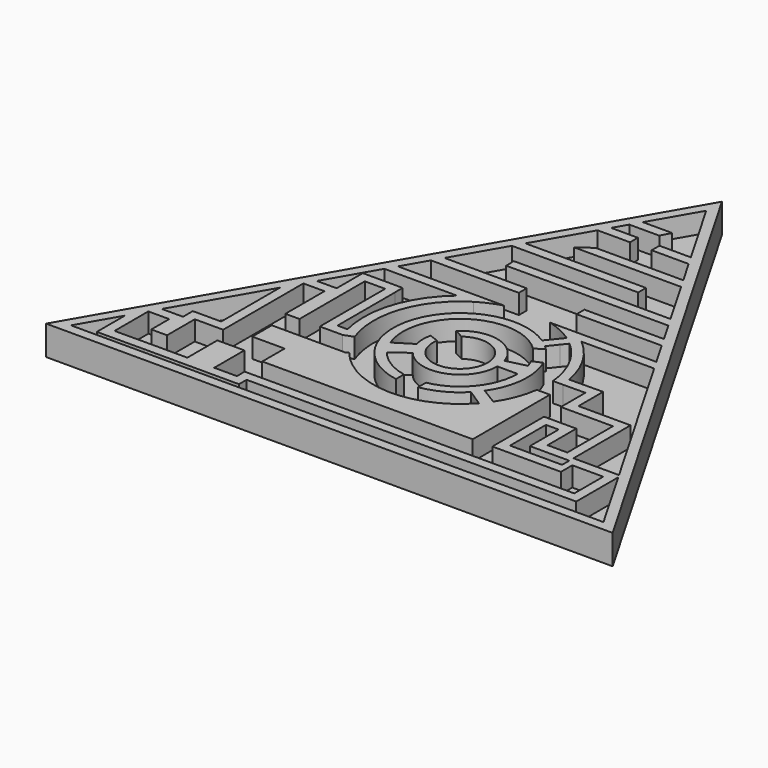
from build123d import *

# Parameters (mm, degrees)
F1_DEPTH = 4
F3_DEPTH = 2


# Not quite as in the source:
# - ends of sketch curves that miss each other by under 0.0002 mm in the source are joined


with BuildPart() as f1:
    # F0 (on Top) → F1 (new body)
    with BuildSketch(Plane.XY):
        Polygon((57.7278355129, -33.3416372538), (0, 66.6583627462), (-57.7278355129, -33.3416372538), align=None)
        Polygon((-36.4066096967, -6.9060390815), (-36.4066096967, -13.5858934373), (-36.4066096967, -15.3864606768), (-40.186252445, -15.3864606768), (-42.186252445, -15.3864606768), (-42.186252445, -17.3864606768), (-42.186252445, -17.8865476996), (-43.4002317488, -17.8865476996), (-46.4966176706, -17.8865476996), (-36.4066096967, -0.4079641283), align=None, mode=Mode.SUBTRACT)
        with BuildLine():
            Line((-27.4925772248, 15.0335163855), (-26.3380205146, 15.0335163855))
            Line((-26.3380205146, 15.0335163855), (-12.690151286, 15.0335163855))
            ThreePointArc((-12.690151286, 15.0335163855), (-18.7426502915, 5.9799343329), (-19.0519640748, -4.9060390815))
            Line((-19.0519640748, -4.9060390815), (-21.0900533497, -4.9060390815))
            Line((-21.0900533497, -4.9060390815), (-21.0900533497, 9.7259394825))
            Line((-21.0900533497, 9.7259394825), (-21.1140420288, 9.7259394825))
            Line((-21.1140420288, 9.7259394825), (-21.1140420288, 11.7116095498))
            Line((-21.1140420288, 11.7116095498), (-23.0900533497, 11.7116095498))
            Line((-23.0900533497, 11.7116095498), (-23.0900533497, 11.7259394825))
            Line((-23.0900533497, 11.7259394825), (-27.2341445088, 11.7259394825))
            Line((-27.2341445088, 11.7259394825), (-29.2341445088, 11.7259394825))
            Line((-29.2341445088, 11.7259394825), (-29.2341445088, 9.7259394825))
            Line((-29.2341445088, 9.7259394825), (-29.2341445088, 5.0565690249))
            Line((-29.2341445088, 5.0565690249), (-30.1103927195, 5.0565690249))
            Line((-30.1103927195, 5.0565690249), (-33.2520529864, 5.0565690249))
            Line((-33.2520529864, 5.0565690249), (-27.4925772248, 15.0335163855))
        make_face(mode=Mode.SUBTRACT)
        Polygon((54.2639496366, -31.3416372538), (-54.2639496366, -31.3416372538), (-49.6511743809, -23.3510808528), (-49.6511743809, -24.4550537318), (-49.6511743809, -28.5100210458), (-49.6511743809, -30.5099894606), (-47.6399342756, -30.5099894606), (-40.0851143612, -30.4675303044), (-40.0738744334, -30.4674671345), (-32.8411310911, -30.4674987197), (-27.3643452674, -30.4674987197), (-20.8822563291, -30.4674987197), (-20.7181237638, -30.4674987197), (-20.7181237638, -28.5053253174), (-20.7108877152, -28.525368914), (-12.9712559283, -28.525368914), (18.1306451559, -28.525368914), (46.4564595819, -28.525368914), (46.4564595819, -26.525368914), (46.4564595819, -19.1514473408), (46.4564595819, -17.8169831846), align=None, mode=Mode.SUBTRACT)
        Polygon((26.1836768538, -20.0500268042), (26.1836768538, -10.8962344453), (28.761634931, -10.8962344453), (28.761634931, -16.2106864154), (28.761634931, -18.2106864154), (30.761634931, -18.2106864154), (34.7944386303, -18.2106864154), (36.7944386303, -18.2106864154), (36.7944386303, -20.0500268042), align=None, mode=Mode.SUBTRACT)
        with BuildLine():
            ThreePointArc((19.3406121337, 3.6037864629), (17.0044739065, 9.8941609921), (12.690151286, 15.0335163855))
            Line((12.690151286, 15.0335163855), (26.3380205146, 15.0335163855))
            Line((26.3380205146, 15.0335163855), (27.4925772248, 15.0335163855))
            Line((27.4925772248, 15.0335163855), (46.0722601447, -17.1514473408))
            Line((46.0722601447, -17.1514473408), (44.4564595819, -17.1514473408))
            Line((44.4564595819, -17.1514473408), (38.1584949791, -17.1514473408))
            Line((38.1584949791, -17.1514473408), (36.7944386303, -17.1514473408))
            Line((36.7944386303, -17.1514473408), (36.7944386303, -16.2106864154))
            Line((36.7944386303, -16.2106864154), (36.7944386303, -8.8962344453))
            Line((36.7944386303, -8.8962344453), (36.7944386303, -2.6055312268))
            Line((36.7944386303, -2.6055312268), (26.1836768538, -2.6055312268))
            Line((26.1836768538, -2.6055312268), (26.1836768538, 3.6767962217))
            Line((26.1836768538, 3.6767962217), (19.456515533, 3.6019981121))
            Line((19.456515533, 3.6019981121), (19.3409452762, 3.6019981121))
            ThreePointArc((19.3409452762, 3.6019981121), (19.3407787256, 3.6028922914), (19.3406121337, 3.6037864629))
        make_face(mode=Mode.SUBTRACT)
        with BuildLine():
            Line((-5.4116371698, 53.2835908234), (0, 62.6579890175))
            Line((0, 62.6579890175), (8.1201158924, 48.5917836587))
            Line((8.1201158924, 48.5917836588), (1.7250510864, 48.5917836588))
            Line((1.7250510864, 48.5917836588), (1.7250510864, 46.5917824588))
            Line((1.7250510864, 46.5917824588), (8.1201158924, 46.5917824588))
            Line((8.1201158924, 46.5917824588), (9.2746732954, 46.5917824588))
            Line((9.2746732954, 46.5917824587), (12.115224579, 41.6711904109))
            Line((12.115224579, 41.6711904109), (-5.7159573771, 41.6711904109))
            Line((-5.7159573771, 41.6711904109), (-8.5862353444, 39.6711895109))
            Line((-8.5862353444, 39.6711895109), (12.0601376528, 39.6711895109))
            Line((12.0601376528, 39.6711895109), (13.2697818089, 39.6711895109))
            Line((13.2697818089, 39.6711895109), (18.8652666503, 29.9783181399))
            Line((18.8652666503, 29.9783181399), (-13.0685195327, 29.9783181399))
            Line((-13.0685195327, 29.9783181399), (-13.0114983767, 27.9783181399))
            Line((-13.0114983767, 27.9783181399), (18.7051940445, 27.9783181399))
            Line((18.7051940445, 27.9783181399), (20.0198233606, 27.9783181399))
            Line((20.0198233606, 27.9783181399), (22.353366566, 23.9359992401))
            Line((22.353366566, 23.9359992401), (6.1596790329, 23.9359992401))
            Line((6.1596790329, 23.9359992401), (6.1596790329, 21.9359992401))
            Line((6.1596790329, 21.9359992401), (22.353366566, 21.9359992401))
            Line((22.353366566, 21.9359992401), (23.5079232763, 21.9359992401))
            Line((23.5079232763, 21.9359992401), (26.3380205146, 17.0335163855))
            Line((26.3380205146, 17.0335163855), (4.7129480122, 17.0335163855))
            ThreePointArc((4.7129480122, 17.0335163855), (7.0736416236, 16.1961771293), (9.2922518534, 15.0335163855))
            ThreePointArc((9.2922518534, 15.0335163855), (9.6774273434, 14.7885076811), (10.056146432, 14.5336326622))
            Line((10.056146432, 14.5336326622), (7.5240175772, 11.4172557392))
            ThreePointArc((7.5240175772, 11.4172557392), (-12.7159372706, 5.0268785987), (-2.3167349644, -13.4758045482))
            Line((-2.3167349644, -13.4758045482), (-2.3152558847, -11.4415979719))
            ThreePointArc((-2.3152558847, -11.4415979719), (-6.1405621571, -9.9279439139), (-9.203241639, -7.1812893896))
            Line((-9.203241639, -7.1812893896), (-5.8634711149, -4.7706568588))
            ThreePointArc((-5.8634711149, -4.7706568588), (2.5315116408, -7.1225633864), (7.5590647821, 0))
            Line((7.5590647821, 0), (11.6734987884, 0))
            ThreePointArc((11.6734987884, 0), (8.9958229761, -7.4394719533), (2.191210068, -11.4660007151))
            Line((2.191210068, -11.4660007151), (2.1897333034, -13.4970232709))
            ThreePointArc((2.1897333034, -13.4970232709), (6.3235444324, -12.1234217499), (9.8155742521, -9.5194049823))
            Line((9.8155742521, -9.5194049823), (13.1991389813, -11.7530970205))
            ThreePointArc((13.1991389813, -11.7530970205), (-0.5179388282, -17.6659078112), (-13.8650427815, -10.9596144134))
            Line((-13.8650427815, -10.9596144134), (-14.3946799421, -11.3673489541))
            Line((-14.3946799421, -11.3673489541), (-20.7108877152, -11.3673489541))
            Line((-20.7108877152, -11.3673489541), (-24.6153641492, -11.3673489541))
            Line((-24.6153641492, -11.3673489541), (-29.3083097786, -11.3673489541))
            Line((-29.3083097786, -11.3673489541), (-29.3083097786, -16.3472294807))
            Line((-29.3083097786, -16.3472294807), (-22.7108877152, -16.3472294807))
            Line((-22.7108877152, -16.3472294807), (-22.7108877152, -20.7385495305))
            Line((-22.7108877152, -20.7385495305), (-22.7108877152, -22.0500268042))
            Line((-22.7108877152, -22.0500268042), (-20.7108877152, -22.0500268042))
            Line((-20.7108877152, -22.0500268042), (-12.685357593, -22.0500268042))
            Line((-12.685357593, -22.0500268042), (18.1306451559, -22.0500268042))
            Line((18.1306451559, -22.0500268042), (20.1836768538, -22.0500268042))
            Line((20.1836768538, -22.0500268042), (20.1836768538, -20.0500268042))
            Line((20.1836768538, -20.0500268042), (20.1836768538, -6.7999763414))
            Line((20.1836768538, -6.7999763414), (20.1836768538, -2.3902875837))
            Line((20.1836768538, -2.3902875837), (19.5268562146, -2.3975906555))
            ThreePointArc((19.5268562146, -2.3975906555), (19.527304214, -2.3939391614), (19.5277515306, -2.3902875837))
            Line((19.5277515306, -2.3902875837), (17.5111131768, -2.3902875837))
            ThreePointArc((17.5111131768, -2.3902875837), (16.5106278722, -6.3048970402), (14.6472129356, -9.8899804166))
            Line((14.6472129356, -9.8899804166), (11.2308936219, -7.7994613641))
            ThreePointArc((11.2308936219, -7.7994613641), (13.6120470756, -1.2948913186), (12.5000423883, 5.5419770305))
            Line((12.5000423883, 5.5419770305), (10.6466540579, 4.7874138459))
            ThreePointArc((10.6466540579, 4.7874138459), (10.9656863196, 4.0030360354), (11.2270192021, 3.1975950021))
            Line((11.2270192021, 3.1975950021), (7.2250536323, 2.2221746987))
            ThreePointArc((7.2250536323, 2.2221746987), (1.9112973644, 7.3134398723), (-5.2139934425, 5.4730003437))
            Line((-5.2139934425, 5.4730003437), (-3.320706901, 4.4582627703))
            ThreePointArc((-3.320706901, 4.4582627703), (4.7345248902, -2.9133271901), (-5.4764306077, 0.9549392919))
            Line((-5.4764306077, 0.9549392919), (-7.3781260289, 1.6439941246))
            ThreePointArc((-7.3781260289, 1.6439941246), (-7.5570187768, -0.1758624105), (-7.2936643109, -1.9854272336))
            Line((-7.2936643109, -1.9854272336), (-10.8843820021, -4.2190997137))
            ThreePointArc((-10.8843820021, -4.2190997137), (-6.4477849908, 9.7312199993), (8.1283956412, 8.3785296002))
            Line((8.1283956412, 8.3785296002), (9.9110118094, 9.4200007447))
            ThreePointArc((9.9110118094, 9.4200007447), (9.5280765896, 9.807156857), (9.1300296654, 10.1787586386))
            Line((9.1300296654, 10.1787586386), (10.6693310663, 12.1167348698))
            Line((10.6693310663, 12.1167348698), (11.6341172668, 13.304129992))
            ThreePointArc((11.6341172668, 13.304129992), (15.2583271949, 8.9182963975), (17.3012513057, 3.6082215395))
            ThreePointArc((17.3012513057, 3.6082215395), (17.4762607398, 2.6096531533), (17.6006047018, 1.603519115))
            Line((17.6006047018, 1.603519115), (19.6080379524, 1.6035592386))
            Line((19.6080379524, 1.6035592386), (24.1836768538, 1.6544349532))
            Line((24.1836768538, 1.6544349532), (24.1836768538, -4.6055312268))
            Line((24.1836768538, -4.6055312268), (34.7944386303, -4.6055312268))
            Line((34.7944386303, -4.6055312268), (34.7944386303, -8.8962344453))
            Line((34.7944386303, -8.8962344453), (34.7944386303, -16.2106864154))
            Line((34.7944386303, -16.2106864154), (30.761634931, -16.2106864154))
            Line((30.761634931, -16.2106864154), (30.761634931, -8.8962344453))
            Line((30.761634931, -8.8962344453), (24.1836768538, -8.8962344453))
            Line((24.1836768538, -8.8962344453), (24.1836768538, -20.0500268042))
            Line((24.1836768538, -20.0500268042), (24.180682376, -20.0500268042))
            Line((24.180682376, -20.0500268042), (24.180682376, -22.0500268042))
            Line((24.180682376, -22.0500268042), (38.1584949791, -22.0500268042))
            Line((38.1584949791, -22.0500268042), (38.1584949791, -20.0500268042))
            Line((38.1584949791, -20.0500268042), (38.1584949791, -19.1514473408))
            Line((38.1584949791, -19.1514473408), (44.4564595819, -19.1514473408))
            Line((44.4564595819, -19.1514473408), (44.4564595819, -26.525368914))
            Line((44.4564595819, -26.525368914), (24.4548246264, -26.525368914))
            Line((24.4548246264, -26.525368914), (18.1306451559, -26.525368914))
            Line((18.1306451559, -26.525368914), (-12.9712559283, -26.525368914))
            Line((-12.9712559283, -26.525368914), (-20.7108877152, -26.525368914))
            Line((-20.7108877152, -26.525368914), (-22.7108877152, -26.525368914))
            Line((-22.7108877152, -26.525368914), (-22.7108877152, -28.5053253174))
            Line((-22.7108877152, -28.5053253174), (-27.3277685046, -28.5053253174))
            Line((-27.3277685046, -28.5053253174), (-27.3277685046, -20.8281986415))
            Line((-27.3277685046, -20.8281986415), (-32.8411310911, -20.8281986415))
            Line((-32.8411310911, -20.8281986415), (-32.8411310911, -28.4674987197))
            Line((-32.8411310911, -28.4674987197), (-40.0851145387, -28.4674987197))
            Line((-40.0851145387, -28.4674987197), (-47.6399346306, -28.5099578768))
            Line((-47.6399346306, -28.5099578768), (-47.6511743809, -28.5100210458))
            Line((-47.6511743809, -28.5100210458), (-47.6511743809, -24.4550537318))
            Line((-47.6511743809, -24.4550537318), (-47.6511743809, -19.8865476996))
            Line((-47.6511743809, -19.8865476996), (-43.4002317488, -19.8865476996))
            Line((-43.4002317488, -19.8865476996), (-43.4002317488, -24.4550537318))
            Line((-43.4002317488, -24.4550537318), (-40.186252445, -24.4550537318))
            Line((-40.186252445, -24.4550537318), (-40.186252445, -24.1824295372))
            Line((-40.186252445, -24.1824295372), (-40.186252445, -17.3864606768))
            Line((-40.186252445, -17.3864606768), (-34.4066096967, -17.3864606768))
            Line((-34.4066096967, -17.3864606768), (-34.4066096967, -13.5858934373))
            Line((-34.4066096967, -13.5858934373), (-34.4066096967, -6.9060390815))
            Line((-34.4066096967, -6.9060390815), (-34.4066096967, 3.0565690249))
            Line((-34.4066096967, 3.0565690249), (-30.1103927195, 3.0565690249))
            Line((-30.1103927195, 3.0565690249), (-30.1103927195, -6.9060390815))
            Line((-30.1103927195, -6.9060390815), (-27.2341445088, -6.9060390815))
            Line((-27.2341445088, -6.9060390815), (-27.2341445088, 9.7259394825))
            Line((-27.2341445088, 9.7259394825), (-23.0900533497, 9.7259394825))
            Line((-23.0900533497, 9.7259394825), (-23.0900533497, -6.9060390815))
            Line((-23.0900533497, -6.9060390815), (-18.4215411619, -6.9060390815))
            Line((-18.4215411619, -6.9060390815), (-16.5441939597, -6.2162855182))
            ThreePointArc((-16.5441939597, -6.2162855182), (-16.7262967599, 5.7082007778), (-9.2922518534, 15.0335163855))
            ThreePointArc((-9.2922518534, 15.0335163855), (-7.0736416236, 16.1961771293), (-4.7129480121, 17.0335163855))
            Line((-4.7129480121, 17.0335163855), (-26.3380205146, 17.0335163855))
            Line((-26.3380205146, 17.0335163855), (-23.5079232763, 21.9359992401))
            Line((-23.5079232763, 21.9359992401), (-22.353366566, 21.9359992401))
            Line((-22.353366566, 21.9359992401), (-5.6064622477, 21.9359992401))
            Line((-5.6064622477, 21.9359992401), (-5.6064622477, 23.9359992401))
            Line((-5.6064622477, 23.9359992401), (-22.353366566, 23.9359992401))
            Line((-22.353366566, 23.9359992401), (-16.5997197009, 33.9028493983))
            Line((-16.5997197009, 33.9028493983), (-15.4451629906, 33.9028493983))
            Line((-15.4451629906, 33.9028493983), (9.1336630285, 33.9028493983))
            Line((9.1336630285, 33.9028493983), (9.1336630285, 35.9028493983))
            Line((9.1336630285, 35.9028493983), (-15.4451629906, 35.9028493983))
            Line((-15.4451629906, 35.9028493983), (-9.2746732954, 46.5917824588))
            Line((-9.2746732954, 46.5917824588), (-8.1201158924, 46.5917824588))
            Line((-8.1201158924, 46.5917824588), (-2.6781822089, 46.5917824588))
            Line((-2.6781822089, 46.5917824588), (-2.6781822089, 48.5917836588))
            Line((-2.6781822089, 48.5917836588), (-8.1201158924, 48.5917836588))
            Line((-8.1201158924, 48.5917836588), (-6.56619388, 51.2835908234))
            Line((-6.56619388, 51.2835908234), (-5.3118569084, 51.2835908234))
            Line((-5.3118569084, 51.2835908234), (-0.4689109046, 51.2835908234))
            Line((-0.4689109046, 51.2835908234), (0.5519921542, 53.2835908234))
            Line((0.5519921542, 53.2835908234), (-5.4116371698, 53.2835908234))
        make_face(mode=Mode.SUBTRACT)
    extrude(amount=F1_DEPTH)

    # F2 (on Top) → F3 (join)
    with BuildSketch(Plane.XY):
        Polygon((-57.7278355129, -33.3416372538), (57.7278355129, -33.3416372538), (0, 66.6583627462), align=None)
    extrude(amount=-F3_DEPTH)


solid = f1.part
